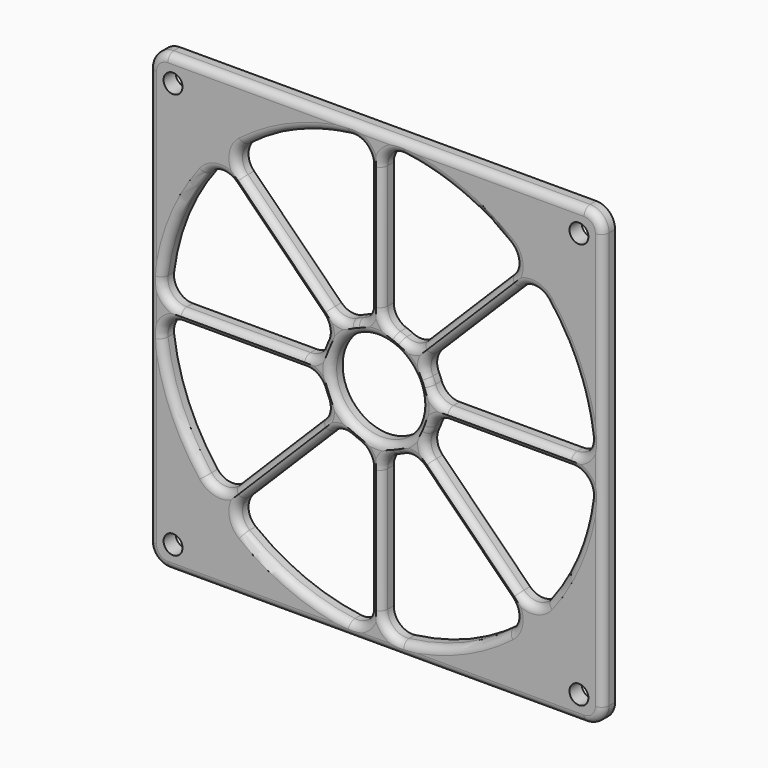
from build123d import *

# Parameters (mm, degrees)
F0_W          = 120
F0_H          = 120
F0_R          = 2.5
F0_R_2        = 12
F1_DEPTH      = 4
F2_R          = 5
F3_T1_DEPTH   = 110
F3_T3_DEPTH   = 110
F3_T5_DEPTH   = 32.6774619337
F3_T7_DEPTH   = 32.6778419819
F3_T9_DEPTH   = 32.6774619337
F3_T11_DEPTH  = 32.6774619337
F3_T13_DEPTH  = 32.6778419819
F3_T15_DEPTH  = 32.6778702464
F3_T17_DEPTH  = 32.677327087
F3_T19_DEPTH  = 32.677327087
F3_T21_DEPTH  = 32.6778419819
F3_T23_DEPTH  = 32.677327087
F3_T25_DEPTH  = 32.6778702464
F3_T27_DEPTH  = 32.677327087
F3_T29_DEPTH  = 32.6778419819
F3_T31_DEPTH  = 32.6778419819
F3_T33_DEPTH  = 32.677327087
F3_T38_ANGLE  = 30.6390253207
F3_T40_ANGLE  = 30.6387768547
F3_T42_ANGLE  = 30.6388811119
F3_T44_ANGLE  = 30.6390253207
F3_T46_ANGLE  = 30.6392737867
F3_T48_ANGLE  = 30.6386326459
F3_T50_ANGLE  = 30.6426556046
F3_T52_ANGLE  = 30.6407162297
F3_T54_ANGLE  = 90
F3_T56_ANGLE  = 90
F3_T58_ANGLE  = 90
F3_T60_ANGLE  = 90
F3_T62_ANGLE  = 97.1806115726
F3_T64_ANGLE  = 97.1786721977
F3_T66_ANGLE  = 71.0401082822
F3_T68_ANGLE  = 7.0749266488
F3_T70_ANGLE  = 71.0348183666
F3_T72_ANGLE  = 97.1786721977
F3_T74_ANGLE  = 97.1786721977
F3_T76_ANGLE  = 71.0401082822
F3_T78_ANGLE  = 7.0802165644
F3_T80_ANGLE  = 71.0401082822
F3_T82_ANGLE  = 97.1807557815
F3_T84_ANGLE  = 97.1806115726
F3_T86_ANGLE  = 71.0348183666
F3_T88_ANGLE  = 7.0692433778
F3_T90_ANGLE  = 71.0344250112
F3_T92_ANGLE  = 97.1779839331
F3_T94_ANGLE  = 97.1779839331
F3_T96_ANGLE  = 71.0419855849
F3_T98_ANGLE  = 7.0792128227
F3_T100_ANGLE = 71.0419855849
F3_T102_ANGLE = 97.1779839331
F3_T104_ANGLE = 97.1806115726
F3_T106_ANGLE = 71.0348183666
F3_T108_ANGLE = 7.074424778
F3_T110_ANGLE = 71.0419855849
F3_T112_ANGLE = 97.1779839331
F3_T114_ANGLE = 97.1807557815
F3_T116_ANGLE = 71.0344250112
F3_T118_ANGLE = 7.0740314225
F3_T120_ANGLE = 71.0419855849
F3_T122_ANGLE = 97.1806115726
F3_T124_ANGLE = 97.1806115726
F3_T126_ANGLE = 71.0348183666
F3_T128_ANGLE = 7.0696367332
F3_T130_ANGLE = 71.0348183666
F3_T132_ANGLE = 97.1779839331
F3_T134_ANGLE = 97.1806115726
F3_T136_ANGLE = 71.0348183666
F3_T138_ANGLE = 7.074424778
F3_T140_ANGLE = 71.0419855849


# Not quite as in the source:
# - a fillet or chamfer that OpenCascade refuses, or shapes differently, is made with other operations: its cross-section is extruded or revolved along the edge and cut away or added


with BuildPart() as f1:
    # F0 (on Front) → F1 (new body)
    with BuildSketch(Plane.XZ):
        Rectangle(F0_W, F0_H)
        with Locations((-53.6360389693, -53.6360389693)):
            Circle(F0_R, mode=Mode.SUBTRACT)
        with Locations((53.6360389693, -53.6360389693)):
            Circle(F0_R, mode=Mode.SUBTRACT)
        with Locations((-53.6360389693, 53.6360389693)):
            Circle(F0_R, mode=Mode.SUBTRACT)
        with BuildLine():
            ThreePointArc((56.9802597397, 1.5), (56.9950647213, 0.7500649435), (57, 0))
            ThreePointArc((57, 0), (56.9950655759, -0.75), (56.9802631579, -1.4998701467))
            ThreePointArc((56.9802631579, -1.4998701467), (52.6611333531, -21.8129556448), (41.3516988244, -39.2305621211))
            ThreePointArc((41.3516988244, -39.2305621211), (40.3050865276, -40.3050865276), (39.2305621211, -41.3516988244))
            ThreePointArc((39.2305621211, -41.3516988244), (21.8129556448, -52.6611333531), (1.4998701467, -56.9802631579))
            ThreePointArc((1.4998701467, -56.9802631579), (0.75, -56.9950655759), (0, -57))
            ThreePointArc((0, -57), (-0.75, -56.9950655759), (-1.4998701467, -56.9802631579))
            ThreePointArc((-1.4998701467, -56.9802631579), (-21.813762616, -52.6607990875), (-39.231829441, -41.3504964748))
            ThreePointArc((-39.231829441, -41.3504964748), (-40.3050865276, -40.3050865276), (-41.3504964748, -39.231829441))
            ThreePointArc((-41.3504964748, -39.231829441), (-52.6611333531, -21.8129556448), (-56.9803090988, -1.4981238267))
            ThreePointArc((-56.9803090988, -1.4981238267), (-56.9950770621, -0.7491266134), (-57, 0))
            ThreePointArc((-57, 0), (-56.9950647213, 0.7500649435), (-56.9802597397, 1.5))
            ThreePointArc((-56.9802597397, 1.5), (-52.6611084982, 21.81301565), (-41.3516988244, 39.2305621211))
            ThreePointArc((-41.3516988244, 39.2305621211), (-40.3050865276, 40.3050865276), (-39.2305621211, 41.3516988244))
            ThreePointArc((-39.2305621211, 41.3516988244), (-21.8129556448, 52.6611333531), (-1.4998701467, 56.9802631579))
            ThreePointArc((-1.4998701467, 56.9802631579), (-0.75, 56.9950655759), (0, 57))
            ThreePointArc((0, 57), (0.75, 56.9950655759), (1.4998701467, 56.9802631579))
            ThreePointArc((1.4998701467, 56.9802631579), (21.8129556448, 52.6611333531), (39.2305621211, 41.3516988244))
            ThreePointArc((39.2305621211, 41.3516988244), (40.3050865276, 40.3050865276), (41.3516988244, 39.2305621211))
            ThreePointArc((41.3516988244, 39.2305621211), (52.6611084982, 21.81301565), (56.9802597397, 1.5))
        make_face(mode=Mode.SUBTRACT)
        with Locations((53.6360389693, 53.6360389693)):
            Circle(F0_R, mode=Mode.SUBTRACT)
        with BuildLine():
            Line((-9.4942351923, 11.6129022261), (-39.2305621211, 41.3516988244))
            ThreePointArc((-39.2305621211, 41.3516988244), (-40.3050865276, 40.3050865276), (-41.3516988244, 39.2305621211))
            Line((-41.3516988244, 39.2305621211), (-11.6140130391, 9.4928763358))
            ThreePointArc((-11.6140130391, 9.4928763358), (-10.6072222233, 10.605981176), (-9.4942351923, 11.6129022261))
        make_face()
        with BuildLine():
            Line((11.6129022261, 9.4942351923), (41.3516988244, 39.2305621211))
            ThreePointArc((41.3516988244, 39.2305621211), (40.3050865276, 40.3050865276), (39.2305621211, 41.3516988244))
            Line((39.2305621211, 41.3516988244), (9.4928763358, 11.6140130391))
            ThreePointArc((9.4928763358, 11.6140130391), (10.605981176, 10.6072222233), (11.6129022261, 9.4942351923))
        make_face()
        with BuildLine():
            Line((0, 15), (0, 57))
            ThreePointArc((0, 57), (-0.75, 56.9950655759), (-1.4998701467, 56.9802631579))
            Line((-1.4998701467, 56.9802631579), (-1.4981238267, 14.925))
            ThreePointArc((-1.4981238267, 14.925), (-0.75, 14.9812382666), (0, 15))
        make_face()
        with BuildLine():
            Line((1.4981238267, 14.925), (1.4998701467, 56.9802631579))
            ThreePointArc((1.4998701467, 56.9802631579), (0.75, 56.9950655759), (0, 57))
            Line((0, 57), (0, 15))
            ThreePointArc((0, 15), (0.75, 14.9812382666), (1.4981238267, 14.925))
        make_face()
        with BuildLine():
            ThreePointArc((14.9248246068, -1.4998701467), (14.9811943633, -0.750876454), (15, 0))
            ThreePointArc((15, 0), (14.9811910967, 0.7509416259), (14.9248115566, 1.5))
            ThreePointArc((14.9248115566, 1.5), (13.8578321638, 5.7411225139), (11.6129022261, 9.4942351923))
            ThreePointArc((11.6129022261, 9.4942351923), (10.605981176, 10.6072222233), (9.4928763358, 11.6140130391))
            ThreePointArc((9.4928763358, 11.6140130391), (5.7394407225, 13.8585287889), (1.4981238267, 14.925))
            ThreePointArc((1.4981238267, 14.925), (0.75, 14.9812382666), (0, 15))
            ThreePointArc((0, 15), (-0.75, 14.9812382666), (-1.4981238267, 14.925))
            ThreePointArc((-1.4981238267, 14.925), (-5.7402514855, 13.8581929877), (-9.4942351923, 11.6129022261))
            ThreePointArc((-9.4942351923, 11.6129022261), (-10.6072222233, 10.605981176), (-11.6140130391, 9.4928763358))
            ThreePointArc((-11.6140130391, 9.4928763358), (-13.858168016, 5.740311772), (-14.9248115566, 1.5))
            ThreePointArc((-14.9248115566, 1.5), (-14.9811910967, 0.7509416259), (-15, 0))
            ThreePointArc((-15, 0), (-14.9812382666, -0.75), (-14.925, -1.4981238267))
            ThreePointArc((-14.925, -1.4981238267), (-13.8581929877, -5.7402514855), (-11.6129022261, -9.4942351923))
            ThreePointArc((-11.6129022261, -9.4942351923), (-10.6066017178, -10.6066017178), (-9.4942351923, -11.6129022261))
            ThreePointArc((-9.4942351923, -11.6129022261), (-5.7410622288, -13.857857139), (-1.4998701467, -14.9248246068))
            ThreePointArc((-1.4998701467, -14.9248246068), (-0.750876454, -14.9811943633), (0, -15))
            ThreePointArc((0, -15), (0.750876454, -14.9811943633), (1.4998701467, -14.9248246068))
            ThreePointArc((1.4998701467, -14.9248246068), (5.7410622288, -13.857857139), (9.4942351923, -11.6129022261))
            ThreePointArc((9.4942351923, -11.6129022261), (10.6072222233, -10.605981176), (11.6140130391, -9.4928763358))
            ThreePointArc((11.6140130391, -9.4928763358), (13.8581929877, -5.7402514855), (14.9248246068, -1.4998701467))
        make_face()
        Circle(F0_R_2, mode=Mode.SUBTRACT)
        with BuildLine():
            Line((15, 0), (57, 0))
            ThreePointArc((57, 0), (56.9950647213, 0.7500649435), (56.9802597397, 1.5))
            Line((56.9802597397, 1.5), (14.9248115566, 1.5))
            ThreePointArc((14.9248115566, 1.5), (14.9811910967, 0.7509416259), (15, 0))
        make_face()
        with BuildLine():
            ThreePointArc((56.9802631579, -1.4998701467), (56.9950655759, -0.75), (57, 0))
            Line((57, 0), (15, 0))
            ThreePointArc((15, 0), (14.9811943633, -0.750876454), (14.9248246068, -1.4998701467))
            Line((14.9248246068, -1.4998701467), (56.9802631579, -1.4998701467))
        make_face()
        with BuildLine():
            ThreePointArc((39.2305621211, -41.3516988244), (40.3050865276, -40.3050865276), (41.3516988244, -39.2305621211))
            Line((41.3516988244, -39.2305621211), (11.6140130391, -9.4928763358))
            ThreePointArc((11.6140130391, -9.4928763358), (10.6072222233, -10.605981176), (9.4942351923, -11.6129022261))
            Line((9.4942351923, -11.6129022261), (39.2305621211, -41.3516988244))
        make_face()
        with BuildLine():
            ThreePointArc((0, -57), (0.75, -56.9950655759), (1.4998701467, -56.9802631579))
            Line((1.4998701467, -56.9802631579), (1.4998701467, -14.9248246068))
            ThreePointArc((1.4998701467, -14.9248246068), (0.750876454, -14.9811943633), (0, -15))
            Line((0, -15), (0, -57))
        make_face()
        with BuildLine():
            ThreePointArc((-1.4998701467, -56.9802631579), (-0.75, -56.9950655759), (0, -57))
            Line((0, -57), (0, -15))
            ThreePointArc((0, -15), (-0.750876454, -14.9811943633), (-1.4998701467, -14.9248246068))
            Line((-1.4998701467, -14.9248246068), (-1.4998701467, -56.9802631579))
        make_face()
        with BuildLine():
            ThreePointArc((-41.3504964748, -39.231829441), (-40.3050865276, -40.3050865276), (-39.231829441, -41.3504964748))
            Line((-39.231829441, -41.3504964748), (-9.4942351923, -11.6129022261))
            ThreePointArc((-9.4942351923, -11.6129022261), (-10.6066017178, -10.6066017178), (-11.6129022261, -9.4942351923))
            Line((-11.6129022261, -9.4942351923), (-41.3504964748, -39.231829441))
        make_face()
        with BuildLine():
            ThreePointArc((-57, 0), (-56.9950770621, -0.7491266134), (-56.9803090988, -1.4981238267))
            Line((-56.9803090988, -1.4981238267), (-14.925, -1.4981238267))
            ThreePointArc((-14.925, -1.4981238267), (-14.9812382666, -0.75), (-15, 0))
            Line((-15, 0), (-57, 0))
        make_face()
        with BuildLine():
            Line((-14.9248115566, 1.5), (-56.9802597397, 1.5))
            ThreePointArc((-56.9802597397, 1.5), (-56.9950647213, 0.7500649435), (-57, 0))
            Line((-57, 0), (-15, 0))
            ThreePointArc((-15, 0), (-14.9811910967, 0.7509416259), (-14.9248115566, 1.5))
        make_face()
    extrude(amount=F1_DEPTH)

    # F2
    f2_edges = [f1.edges().sort_by_distance(p)[0] for p in [
        (-60, -2, 60),
        (60, -2, 60),
        (60, -2, -60),
        (-60, -2, -60),
        (-14.924812, -2, 1.5),
        (-11.614013, -2, 9.492876),
        (-9.494235, -2, 11.612902),
        (-1.498124, -2, 14.925),
        (-39.230562, -2, 41.351699),
        (-41.351699, -2, 39.230562),
        (-56.98026, -2, 1.5),
        (-56.980309, -2, -1.498124),
        (-41.350496, -2, -39.231829),
        (-14.925, -2, -1.498124),
        (-11.612902, -2, -9.494235),
        (-9.494235, -2, -11.612902),
        (-39.231829, -2, -41.350496),
        (-1.49987, -2, -56.980263),
        (-1.49987, -2, -14.924825),
        (1.49987, -2, -14.924825),
        (1.49987, -2, -56.980263),
        (39.230562, -2, -41.351699),
        (9.494235, -2, -11.612902),
        (11.614013, -2, -9.492876),
        (41.351699, -2, -39.230562),
        (56.980263, -2, -1.49987),
        (14.924825, -2, -1.49987),
        (14.924812, -2, 1.5),
        (56.98026, -2, 1.5),
        (41.351699, -2, 39.230562),
        (11.612902, -2, 9.494235),
        (9.492876, -2, 11.614013),
        (1.498124, -2, 14.925),
        (39.230562, -2, 41.351699),
        (1.49987, -2, 56.980263),
        (-1.49987, -2, 56.980263),
    ]]
    fillet(f2_edges, radius=F2_R)

    # F3: fillet of radius 2 on 10 edges, made by hand

    # F3_s2 → F3_t1 (cut)
    with BuildSketch(Plane.YZ.offset(-55)):
        with BuildLine():
            ThreePointArc((-2, 60), (-3.4142135624, 59.4142135624), (-4, 58))
            Line((-4, 58), (-4.04, 58))
            Line((-4.04, 58), (-4.04, 60.04))
            Line((-4.04, 60.04), (-2, 60.04))
            Line((-2, 60.04), (-2, 60))
        make_face()
        with BuildLine():
            ThreePointArc((-4, -58), (-3.4142135624, -59.4142135624), (-2, -60))
            Line((-2, -60), (-2, -60.04))
            Line((-2, -60.04), (-4.04, -60.04))
            Line((-4.04, -60.04), (-4.04, -58))
            Line((-4.04, -58), (-4, -58))
        make_face()
    extrude(amount=F3_T1_DEPTH, mode=Mode.SUBTRACT)

    # F3_s4 → F3_t3 (cut)
    with BuildSketch(Plane.XY.offset(-55)):
        with BuildLine():
            ThreePointArc((-58, -4), (-59.4142135624, -3.4142135624), (-60, -2))
            Line((-60, -2), (-60.04, -2))
            Line((-60.04, -2), (-60.04, -4.04))
            Line((-60.04, -4.04), (-58, -4.04))
            Line((-58, -4.04), (-58, -4))
        make_face()
        with BuildLine():
            ThreePointArc((58, -4), (59.4142135624, -3.4142135624), (60, -2))
            Line((60, -2), (60.04, -2))
            Line((60.04, -2), (60.04, -4.04))
            Line((60.04, -4.04), (58, -4.04))
            Line((58, -4.04), (58, -4))
        make_face()
    extrude(amount=F3_T3_DEPTH, mode=Mode.SUBTRACT)

    # F3_s6 → F3_t5 (cut)
    with BuildSketch(Plane(origin=(-36.4813266393, 0, -36.4813266393), x_dir=(0, 1, 0), z_dir=(0.7071067812, 0, 0.7071067812))):
        with BuildLine():
            ThreePointArc((-4, 0.5018761733), (-3.4142135624, -0.912337389), (-2, -1.4981238267))
            Line((-2, -1.4981238267), (-2, -1.5381238267))
            Line((-2, -1.5381238267), (-4.04, -1.5381238267))
            Line((-4.04, -1.5381238267), (-4.04, 0.5018761733))
            Line((-4.04, 0.5018761733), (-4, 0.5018761733))
        make_face()
    extrude(amount=F3_T5_DEPTH, mode=Mode.SUBTRACT)

    # F3_s8 → F3_t7 (cut)
    with BuildSketch(Plane.XY.offset(-51.5921669256)):
        with BuildLine():
            ThreePointArc((0.5001298533, -4), (-0.9140837091, -3.4142135624), (-1.4998701467, -2))
            Line((-1.4998701467, -2), (-1.5398701467, -2))
            Line((-1.5398701467, -2), (-1.5398701467, -4.04))
            Line((-1.5398701467, -4.04), (0.5001298533, -4.04))
            Line((0.5001298533, -4.04), (0.5001298533, -4))
        make_face()
        with BuildLine():
            ThreePointArc((-0.5001298533, -4), (0.9140837091, -3.4142135624), (1.4998701467, -2))
            Line((1.4998701467, -2), (1.5398701467, -2))
            Line((1.5398701467, -2), (1.5398701467, -4.04))
            Line((1.5398701467, -4.04), (-0.5001298533, -4.04))
            Line((-0.5001298533, -4.04), (-0.5001298533, -4))
        make_face()
    extrude(amount=F3_T7_DEPTH, mode=Mode.SUBTRACT)

    # F3_s10 → F3_t9 (cut)
    with BuildSketch(Plane.YZ.offset(-51.5923869067)):
        with BuildLine():
            ThreePointArc((-4, 0.5018761733), (-3.4142135624, -0.912337389), (-2, -1.4981238267))
            Line((-2, -1.4981238267), (-2, -1.5381238267))
            Line((-2, -1.5381238267), (-4.04, -1.5381238267))
            Line((-4.04, -1.5381238267), (-4.04, 0.5018761733))
            Line((-4.04, 0.5018761733), (-4, 0.5018761733))
        make_face()
    extrude(amount=F3_T9_DEPTH, mode=Mode.SUBTRACT)

    # F3_s12 → F3_t11 (cut)
    with BuildSketch(Plane(origin=(-13.374871714, 0, -13.374871714), x_dir=(0, 1, 0), z_dir=(-0.7071067812, 0, -0.7071067812))):
        with BuildLine():
            ThreePointArc((-4, 0.5018761733), (-3.4142135624, -0.912337389), (-2, -1.4981238267))
            Line((-2, -1.4981238267), (-2, -1.5381238267))
            Line((-2, -1.5381238267), (-4.04, -1.5381238267))
            Line((-4.04, -1.5381238267), (-4.04, 0.5018761733))
            Line((-4.04, 0.5018761733), (-4, 0.5018761733))
        make_face()
    extrude(amount=F3_T11_DEPTH, mode=Mode.SUBTRACT)

    # F3_s14 → F3_t13 (cut)
    with BuildSketch(Plane(origin=(-36.4811710892, 0, 36.4811710892), x_dir=(0, 1, 0), z_dir=(0.7071067812, 0, -0.7071067812))):
        with BuildLine():
            ThreePointArc((-4, 0.5001298533), (-3.4142135624, -0.9140837091), (-2, -1.4998701467))
            Line((-2, -1.4998701467), (-2, -1.5398701467))
            Line((-2, -1.5398701467), (-4.04, -1.5398701467))
            Line((-4.04, -1.5398701467), (-4.04, 0.5001298533))
            Line((-4.04, 0.5001298533), (-4, 0.5001298533))
        make_face()
    extrude(amount=F3_T13_DEPTH, mode=Mode.SUBTRACT)

    # F3_s16 → F3_t15 (cut)
    with BuildSketch(Plane.YZ.offset(-51.5921505658)):
        with BuildLine():
            ThreePointArc((-4, -0.5), (-3.4142135624, 0.9142135624), (-2, 1.5))
            Line((-2, 1.5), (-2, 1.54))
            Line((-2, 1.54), (-4.04, 1.54))
            Line((-4.04, 1.54), (-4.04, -0.5))
            Line((-4.04, -0.5), (-4, -0.5))
        make_face()
    extrude(amount=F3_T15_DEPTH, mode=Mode.SUBTRACT)

    # F3_s18 → F3_t17 (cut)
    with BuildSketch(Plane(origin=(-0.0021423468, 0, 51.5924649171), x_dir=(0, 1, 0), z_dir=(4.15244e-05, 0, -0.9999999991))):
        with BuildLine():
            ThreePointArc((-4, 0.5024959265), (-3.4142135624, -0.9117176359), (-2, -1.4975040735))
            Line((-2, -1.4975040735), (-2, -1.5375040735))
            Line((-2, -1.5375040735), (-4.04, -1.5375040735))
            Line((-4.04, -1.5375040735), (-4.04, 0.5024959265))
            Line((-4.04, 0.5024959265), (-4, 0.5024959265))
        make_face()
    extrude(amount=F3_T17_DEPTH, mode=Mode.SUBTRACT)

    # F3_s20 → F3_t19 (cut)
    with BuildSketch(Plane(origin=(-13.3744668567, 0, 13.3755776366), x_dir=(0, 1, 0), z_dir=(-0.7070774184, 0, 0.7071361428))):
        with BuildLine():
            ThreePointArc((-4, 0.5024959265), (-3.4142135624, -0.9117176359), (-2, -1.4975040735))
            Line((-2, -1.4975040735), (-2, -1.5375040735))
            Line((-2, -1.5375040735), (-4.04, -1.5375040735))
            Line((-4.04, -1.5375040735), (-4.04, 0.5024959265))
            Line((-4.04, 0.5024959265), (-4, 0.5024959265))
        make_face()
    extrude(amount=F3_T19_DEPTH, mode=Mode.SUBTRACT)

    # F3_s22 → F3_t21 (cut)
    with BuildSketch(Plane(origin=(36.4811710892, 0, 36.4811710892), x_dir=(0, 1, 0), z_dir=(-0.7071067812, 0, -0.7071067812))):
        with BuildLine():
            ThreePointArc((-4, 0.5001298533), (-3.4142135624, -0.9140837091), (-2, -1.4998701467))
            Line((-2, -1.4998701467), (-2, -1.5398701467))
            Line((-2, -1.5398701467), (-4.04, -1.5398701467))
            Line((-4.04, -1.5398701467), (-4.04, 0.5001298533))
            Line((-4.04, 0.5001298533), (-4, 0.5001298533))
        make_face()
    extrude(amount=F3_T21_DEPTH, mode=Mode.SUBTRACT)

    # F3_s24 → F3_t23 (cut)
    with BuildSketch(Plane(origin=(0.00078544, 0, 18.9151378583), x_dir=(0, 1, 0), z_dir=(4.15244e-05, 0, 0.9999999991))):
        with BuildLine():
            ThreePointArc((-4, 0.5024959265), (-3.4142135624, -0.9117176359), (-2, -1.4975040735))
            Line((-2, -1.4975040735), (-2, -1.5375040735))
            Line((-2, -1.5375040735), (-4.04, -1.5375040735))
            Line((-4.04, -1.5375040735), (-4.04, 0.5024959265))
            Line((-4.04, 0.5024959265), (-4, 0.5024959265))
        make_face()
    extrude(amount=F3_T23_DEPTH, mode=Mode.SUBTRACT)

    # F3_s26 → F3_t25 (cut)
    with BuildSketch(Plane.YZ.offset(18.9142803194)):
        with BuildLine():
            ThreePointArc((-4, -0.5), (-3.4142135624, 0.9142135624), (-2, 1.5))
            Line((-2, 1.5), (-2, 1.54))
            Line((-2, 1.54), (-4.04, 1.54))
            Line((-4.04, 1.54), (-4.04, -0.5))
            Line((-4.04, -0.5), (-4, -0.5))
        make_face()
    extrude(amount=F3_T25_DEPTH, mode=Mode.SUBTRACT)

    # F3_s28 → F3_t27 (cut)
    with BuildSketch(Plane(origin=(13.3755776366, 0, 13.3744668567), x_dir=(0, 1, 0), z_dir=(0.7071361428, 0, 0.7070774184))):
        with BuildLine():
            ThreePointArc((-4, 0.5024959265), (-3.4142135624, -0.9117176359), (-2, -1.4975040735))
            Line((-2, -1.4975040735), (-2, -1.5375040735))
            Line((-2, -1.5375040735), (-4.04, -1.5375040735))
            Line((-4.04, -1.5375040735), (-4.04, 0.5024959265))
            Line((-4.04, 0.5024959265), (-4, 0.5024959265))
        make_face()
    extrude(amount=F3_T27_DEPTH, mode=Mode.SUBTRACT)

    # F3_s30 → F3_t29 (cut)
    with BuildSketch(Plane(origin=(36.4811710892, 0, -36.4811710892), x_dir=(0, 1, 0), z_dir=(-0.7071067812, 0, 0.7071067812))):
        with BuildLine():
            ThreePointArc((-4, 0.5001298533), (-3.4142135624, -0.9140837091), (-2, -1.4998701467))
            Line((-2, -1.4998701467), (-2, -1.5398701467))
            Line((-2, -1.5398701467), (-4.04, -1.5398701467))
            Line((-4.04, -1.5398701467), (-4.04, 0.5001298533))
            Line((-4.04, 0.5001298533), (-4, 0.5001298533))
        make_face()
    extrude(amount=F3_T29_DEPTH, mode=Mode.SUBTRACT)

    # F3_s32 → F3_t31 (cut)
    with BuildSketch(Plane.YZ.offset(18.9143249437)):
        with BuildLine():
            ThreePointArc((-4, 0.5001298533), (-3.4142135624, -0.9140837091), (-2, -1.4998701467))
            Line((-2, -1.4998701467), (-2, -1.5398701467))
            Line((-2, -1.5398701467), (-4.04, -1.5398701467))
            Line((-4.04, -1.5398701467), (-4.04, 0.5001298533))
            Line((-4.04, 0.5001298533), (-4, 0.5001298533))
        make_face()
    extrude(amount=F3_T31_DEPTH, mode=Mode.SUBTRACT)

    # F3_s34 → F3_t33 (cut)
    with BuildSketch(Plane(origin=(13.3744668567, 0, -13.3755776366), x_dir=(0, 1, 0), z_dir=(0.7070774184, 0, -0.7071361428))):
        with BuildLine():
            ThreePointArc((-4, 0.5024959265), (-3.4142135624, -0.9117176359), (-2, -1.4975040735))
            Line((-2, -1.4975040735), (-2, -1.5375040735))
            Line((-2, -1.5375040735), (-4.04, -1.5375040735))
            Line((-4.04, -1.5375040735), (-4.04, 0.5024959265))
            Line((-4.04, 0.5024959265), (-4, 0.5024959265))
        make_face()
    extrude(amount=F3_T33_DEPTH, mode=Mode.SUBTRACT)

    # F3_s35 → F3_t36 (revolve, cut)
    with BuildSketch(Plane.XY):
        with BuildLine():
            ThreePointArc((14, -4), (12.5857864376, -3.4142135624), (12, -2))
            Line((12, -2), (11.96, -2))
            Line((11.96, -2), (11.96, -4.04))
            Line((11.96, -4.04), (14, -4.04))
            Line((14, -4.04), (14, -4))
        make_face()
    revolve(axis=Axis((0, -4, 0), (0, -1, 0)), mode=Mode.SUBTRACT)

    # F3_s37 → F3_t38 (revolve, cut)
    with BuildSketch(Plane(origin=(0, 0, 0), x_dir=(0, 1, 0), z_dir=(0.7899449053, 0, 0.6131778262))):
        with BuildLine():
            ThreePointArc((-4, -59), (-3.4142135624, -57.5857864376), (-2, -57))
            Line((-2, -57), (-2, -56.96))
            Line((-2, -56.96), (-4.04, -56.96))
            Line((-4.04, -56.96), (-4.04, -59))
            Line((-4.04, -59), (-4, -59))
        make_face()
    revolve(axis=Axis((0, -4, 0), (0, 1, 0)), revolution_arc=F3_T38_ANGLE, mode=Mode.SUBTRACT)

    # F3_s39 → F3_t40 (revolve, cut)
    with BuildSketch(Plane(origin=(0, 0, 0), x_dir=(0, 1, 0), z_dir=(0.1249975028, 0, 0.9921570563))):
        with BuildLine():
            ThreePointArc((-4, -59), (-3.4142135624, -57.5857864376), (-2, -57))
            Line((-2, -57), (-2, -56.96))
            Line((-2, -56.96), (-4.04, -56.96))
            Line((-4.04, -56.96), (-4.04, -59))
            Line((-4.04, -59), (-4, -59))
        make_face()
    revolve(axis=Axis((0, -4, 0), (0, 1, 0)), revolution_arc=F3_T40_ANGLE, mode=Mode.SUBTRACT)

    # F3_s41 → F3_t42 (revolve, cut)
    with BuildSketch(Plane(origin=(0, 0, 0), x_dir=(0, 1, 0), z_dir=(-0.6131778262, 0, 0.7899449053))):
        with BuildLine():
            ThreePointArc((-4, -59), (-3.4142135624, -57.5857864376), (-2, -57))
            Line((-2, -57), (-2, -56.96))
            Line((-2, -56.96), (-4.04, -56.96))
            Line((-4.04, -56.96), (-4.04, -59))
            Line((-4.04, -59), (-4, -59))
        make_face()
    revolve(axis=Axis((0, -4, 0), (0, 1, 0)), revolution_arc=F3_T42_ANGLE, mode=Mode.SUBTRACT)

    # F3_s43 → F3_t44 (revolve, cut)
    with BuildSketch(Plane(origin=(0, 0, 0), x_dir=(0, 1, 0), z_dir=(-0.9921575983, 0, 0.1249932003))):
        with BuildLine():
            ThreePointArc((-4, -59), (-3.4142135624, -57.5857864376), (-2, -57))
            Line((-2, -57), (-2, -56.96))
            Line((-2, -56.96), (-4.04, -56.96))
            Line((-4.04, -56.96), (-4.04, -59))
            Line((-4.04, -59), (-4, -59))
        make_face()
    revolve(axis=Axis((0, -4, 0), (0, 1, 0)), revolution_arc=F3_T44_ANGLE, mode=Mode.SUBTRACT)

    # F3_s45 → F3_t46 (revolve, cut)
    with BuildSketch(Plane(origin=(0, 0, 0), x_dir=(0, 1, 0), z_dir=(-0.7899449053, 0, -0.6131778262))):
        with BuildLine():
            ThreePointArc((-4, -59), (-3.4142135624, -57.5857864376), (-2, -57))
            Line((-2, -57), (-2, -56.96))
            Line((-2, -56.96), (-4.04, -56.96))
            Line((-4.04, -56.96), (-4.04, -59))
            Line((-4.04, -59), (-4, -59))
        make_face()
    revolve(axis=Axis((0, -4, 0), (0, 1, 0)), revolution_arc=F3_T46_ANGLE, mode=Mode.SUBTRACT)

    # F3_s47 → F3_t48 (revolve, cut)
    with BuildSketch(Plane(origin=(0, 0, 0), x_dir=(0, 1, 0), z_dir=(-0.125, 0, -0.9921567416))):
        with BuildLine():
            ThreePointArc((-4, -59), (-3.4142135624, -57.5857864376), (-2, -57))
            Line((-2, -57), (-2, -56.96))
            Line((-2, -56.96), (-4.04, -56.96))
            Line((-4.04, -56.96), (-4.04, -59))
            Line((-4.04, -59), (-4, -59))
        make_face()
    revolve(axis=Axis((0, -4, 0), (0, 1, 0)), revolution_arc=F3_T48_ANGLE, mode=Mode.SUBTRACT)

    # F3_s49 → F3_t50 (revolve, cut)
    with BuildSketch(Plane(origin=(0, 0, 0), x_dir=(0, 1, 0), z_dir=(0.6132011388, 0, -0.7899268089))):
        with BuildLine():
            ThreePointArc((-4, -59), (-3.4142135624, -57.5857864376), (-2, -57))
            Line((-2, -57), (-2, -56.96))
            Line((-2, -56.96), (-4.04, -56.96))
            Line((-4.04, -56.96), (-4.04, -59))
            Line((-4.04, -59), (-4, -59))
        make_face()
    revolve(axis=Axis((0, -4, 0), (0, 1, 0)), revolution_arc=F3_T50_ANGLE, mode=Mode.SUBTRACT)

    # F3_s51 → F3_t52 (revolve, cut)
    with BuildSketch(Plane(origin=(0, 0, 0), x_dir=(0, 1, 0), z_dir=(0.9921570563, 0, -0.1249975028))):
        with BuildLine():
            ThreePointArc((-4, -59), (-3.4142135624, -57.5857864376), (-2, -57))
            Line((-2, -57), (-2, -56.96))
            Line((-2, -56.96), (-4.04, -56.96))
            Line((-4.04, -56.96), (-4.04, -59))
            Line((-4.04, -59), (-4, -59))
        make_face()
    revolve(axis=Axis((0, -4, 0), (0, 1, 0)), revolution_arc=F3_T52_ANGLE, mode=Mode.SUBTRACT)

    # F3_s53 → F3_t54 (revolve, cut)
    with BuildSketch(Plane.YZ.offset(55)):
        with BuildLine():
            ThreePointArc((-2, 60), (-3.4142135624, 59.4142135624), (-4, 58))
            Line((-4, 58), (-4.04, 58))
            Line((-4.04, 58), (-4.04, 60.04))
            Line((-4.04, 60.04), (-2, 60.04))
            Line((-2, 60.04), (-2, 60))
        make_face()
    revolve(axis=Axis((55, -4, 55), (0, 1, 0)), revolution_arc=F3_T54_ANGLE, mode=Mode.SUBTRACT)

    # F3_s55 → F3_t56 (revolve, cut)
    with BuildSketch(Plane.YZ.offset(-55)):
        with BuildLine():
            ThreePointArc((-2, 60), (-3.4142135624, 59.4142135624), (-4, 58))
            Line((-4, 58), (-4.04, 58))
            Line((-4.04, 58), (-4.04, 60.04))
            Line((-4.04, 60.04), (-2, 60.04))
            Line((-2, 60.04), (-2, 60))
        make_face()
    revolve(axis=Axis((-55, -4, 55), (0, -1, 0)), revolution_arc=F3_T56_ANGLE, mode=Mode.SUBTRACT)

    # F3_s57 → F3_t58 (revolve, cut)
    with BuildSketch(Plane.XY.offset(-55)):
        with BuildLine():
            ThreePointArc((-58, -4), (-59.4142135624, -3.4142135624), (-60, -2))
            Line((-60, -2), (-60.04, -2))
            Line((-60.04, -2), (-60.04, -4.04))
            Line((-60.04, -4.04), (-58, -4.04))
            Line((-58, -4.04), (-58, -4))
        make_face()
    revolve(axis=Axis((-55, -4, -55), (0, -1, 0)), revolution_arc=F3_T58_ANGLE, mode=Mode.SUBTRACT)

    # F3_s59 → F3_t60 (revolve, cut)
    with BuildSketch(Plane.YZ.offset(55)):
        with BuildLine():
            ThreePointArc((-4, -58), (-3.4142135624, -59.4142135624), (-2, -60))
            Line((-2, -60), (-2, -60.04))
            Line((-2, -60.04), (-4.04, -60.04))
            Line((-4.04, -60.04), (-4.04, -58))
            Line((-4.04, -58), (-4, -58))
        make_face()
    revolve(axis=Axis((55, -4, -55), (0, -1, 0)), revolution_arc=F3_T60_ANGLE, mode=Mode.SUBTRACT)

    # F3_s61 → F3_t62 (revolve, cut)
    with BuildSketch(Plane.XY.offset(-51.5921669256)):
        with BuildLine():
            ThreePointArc((0.5001298533, -4), (-0.9140837091, -3.4142135624), (-1.4998701467, -2))
            Line((-1.4998701467, -2), (-1.5398701467, -2))
            Line((-1.5398701467, -2), (-1.5398701467, -4.04))
            Line((-1.5398701467, -4.04), (0.5001298533, -4.04))
            Line((0.5001298533, -4.04), (0.5001298533, -4))
        make_face()
    revolve(axis=Axis((-6.4998701467, -4, -51.5921669256), (0, 1, 0)), revolution_arc=F3_T62_ANGLE, mode=Mode.SUBTRACT)

    # F3_s63 → F3_t64 (revolve, cut)
    with BuildSketch(Plane(origin=(0, 0, 0), x_dir=(0, 1, 0), z_dir=(0.7899268089, 0, -0.6132011388))):
        with BuildLine():
            ThreePointArc((-4, -59), (-3.4142135624, -57.5857864376), (-2, -57))
            Line((-2, -57), (-2, -56.96))
            Line((-2, -56.96), (-4.04, -56.96))
            Line((-4.04, -56.96), (-4.04, -59))
            Line((-4.04, -59), (-4, -59))
        make_face()
    revolve(axis=Axis((-31.8864592165, -4, -41.0761940622), (0, 1, 0)), revolution_arc=F3_T64_ANGLE, mode=Mode.SUBTRACT)

    # F3_s65 → F3_t66 (revolve, cut)
    with BuildSketch(Plane(origin=(0, 0, 0), x_dir=(0, 1, 0), z_dir=(0.8984869568, 0, -0.4390002146))):
        with BuildLine():
            ThreePointArc((-4, -13), (-3.4142135624, -14.4142135624), (-2, -15))
            Line((-2, -15), (-2, -15.04))
            Line((-2, -15.04), (-4.04, -15.04))
            Line((-4.04, -15.04), (-4.04, -13))
            Line((-4.04, -13), (-4, -13))
        make_face()
    revolve(axis=Axis((-8.7800042912, -4, -17.9697391368), (0, -1, 0)), revolution_arc=F3_T66_ANGLE, mode=Mode.SUBTRACT)

    # F3_s67 → F3_t68 (revolve, cut)
    with BuildSketch(Plane(origin=(0, 0, 0), x_dir=(0, 1, 0), z_dir=(-0.8984869568, 0, 0.4390002146))):
        with BuildLine():
            ThreePointArc((-4, 13), (-3.4142135624, 14.4142135624), (-2, 15))
            Line((-2, 15), (-2, 15.04))
            Line((-2, 15.04), (-4.04, 15.04))
            Line((-4.04, 15.04), (-4.04, 13))
            Line((-4.04, 13), (-4, 13))
        make_face()
    revolve(axis=Axis((0, -4, 0), (0, -1, 0)), revolution_arc=F3_T68_ANGLE, mode=Mode.SUBTRACT)

    # F3_s69 → F3_t70 (revolve, cut)
    with BuildSketch(Plane(origin=(0, 0, 0), x_dir=(0, 1, 0), z_dir=(-0.9457162472, 0, 0.3249935073))):
        with BuildLine():
            ThreePointArc((-4, 13), (-3.4142135624, 14.4142135624), (-2, 15))
            Line((-2, 15), (-2, 15.04))
            Line((-2, 15.04), (-4.04, 15.04))
            Line((-4.04, 15.04), (-4.04, 13))
            Line((-4.04, 13), (-4, 13))
        make_face()
    revolve(axis=Axis((-6.4998701467, -4, -18.9143249437), (0, 1, 0)), revolution_arc=F3_T70_ANGLE, mode=Mode.SUBTRACT)

    # F3_s71 → F3_t72 (revolve, cut)
    with BuildSketch(Plane(origin=(-36.4813266393, 0, -36.4813266393), x_dir=(0, 1, 0), z_dir=(0.7071067812, 0, 0.7071067812))):
        with BuildLine():
            ThreePointArc((-4, -0.5018761733), (-3.4142135624, 0.912337389), (-2, 1.4981238267))
            Line((-2, 1.4981238267), (-2, 1.5381238267))
            Line((-2, 1.5381238267), (-4.04, 1.5381238267))
            Line((-4.04, 1.5381238267), (-4.04, -0.5018761733))
            Line((-4.04, -0.5018761733), (-4, -0.5018761733))
        make_face()
    revolve(axis=Axis((-41.0761940622, -4, -31.8864592165), (0, 1, 0)), revolution_arc=F3_T72_ANGLE, mode=Mode.SUBTRACT)

    # F3_s73 → F3_t74 (revolve, cut)
    with BuildSketch(Plane(origin=(0, 0, 0), x_dir=(0, 1, 0), z_dir=(0.1249639197, 0, -0.9921612867))):
        with BuildLine():
            ThreePointArc((-4, -59), (-3.4142135624, -57.5857864376), (-2, -57))
            Line((-2, -57), (-2, -56.96))
            Line((-2, -56.96), (-4.04, -56.96))
            Line((-4.04, -56.96), (-4.04, -59))
            Line((-4.04, -59), (-4, -59))
        make_face()
    revolve(axis=Axis((-51.5923869067, -4, -6.4981238267), (0, 1, 0)), revolution_arc=F3_T74_ANGLE, mode=Mode.SUBTRACT)

    # F3_s75 → F3_t76 (revolve, cut)
    with BuildSketch(Plane(origin=(0, 0, 0), x_dir=(0, 1, 0), z_dir=(0.3249061913, 0, -0.9457462486))):
        with BuildLine():
            ThreePointArc((-4, -13), (-3.4142135624, -14.4142135624), (-2, -15))
            Line((-2, -15), (-2, -15.04))
            Line((-2, -15.04), (-4.04, -15.04))
            Line((-4.04, -15.04), (-4.04, -13))
            Line((-4.04, -13), (-4, -13))
        make_face()
    revolve(axis=Axis((-18.914924973, -4, -6.4981238267), (0, -1, 0)), revolution_arc=F3_T76_ANGLE, mode=Mode.SUBTRACT)

    # F3_s77 → F3_t78 (revolve, cut)
    with BuildSketch(Plane(origin=(0, 0, 0), x_dir=(0, 1, 0), z_dir=(-0.3249061913, 0, 0.9457462486))):
        with BuildLine():
            ThreePointArc((-4, 13), (-3.4142135624, 14.4142135624), (-2, 15))
            Line((-2, 15), (-2, 15.04))
            Line((-2, 15.04), (-4.04, 15.04))
            Line((-4.04, 15.04), (-4.04, 13))
            Line((-4.04, 13), (-4, 13))
        make_face()
    revolve(axis=Axis((0, -4, 0), (0, -1, 0)), revolution_arc=F3_T78_ANGLE, mode=Mode.SUBTRACT)

    # F3_s79 → F3_t80 (revolve, cut)
    with BuildSketch(Plane(origin=(0, 0, 0), x_dir=(0, 1, 0), z_dir=(-0.4390002146, 0, 0.8984869568))):
        with BuildLine():
            ThreePointArc((-4, 13), (-3.4142135624, 14.4142135624), (-2, 15))
            Line((-2, 15), (-2, 15.04))
            Line((-2, 15.04), (-4.04, 15.04))
            Line((-4.04, 15.04), (-4.04, 13))
            Line((-4.04, 13), (-4, 13))
        make_face()
    revolve(axis=Axis((-17.9697391368, -4, -8.7800042912), (0, 1, 0)), revolution_arc=F3_T80_ANGLE, mode=Mode.SUBTRACT)

    # F3_s81 → F3_t82 (revolve, cut)
    with BuildSketch(Plane.YZ.offset(-51.5921505658)):
        with BuildLine():
            ThreePointArc((-4, -0.5), (-3.4142135624, 0.9142135624), (-2, 1.5))
            Line((-2, 1.5), (-2, 1.54))
            Line((-2, 1.54), (-4.04, 1.54))
            Line((-4.04, 1.54), (-4.04, -0.5))
            Line((-4.04, -0.5), (-4, -0.5))
        make_face()
    revolve(axis=Axis((-51.5921505658, -4, 6.5), (0, 1, 0)), revolution_arc=F3_T82_ANGLE, mode=Mode.SUBTRACT)

    # F3_s83 → F3_t84 (revolve, cut)
    with BuildSketch(Plane(origin=(-36.4811710892, 0, 36.4811710892), x_dir=(0, 1, 0), z_dir=(0.7071067812, 0, -0.7071067812))):
        with BuildLine():
            ThreePointArc((-4, 0.5001298533), (-3.4142135624, -0.9140837091), (-2, -1.4998701467))
            Line((-2, -1.4998701467), (-2, -1.5398701467))
            Line((-2, -1.5398701467), (-4.04, -1.5398701467))
            Line((-4.04, -1.5398701467), (-4.04, 0.5001298533))
            Line((-4.04, 0.5001298533), (-4, 0.5001298533))
        make_face()
    revolve(axis=Axis((-41.0772733468, -4, 31.8850688316), (0, -1, 0)), revolution_arc=F3_T84_ANGLE, mode=Mode.SUBTRACT)

    # F3_s85 → F3_t86 (revolve, cut)
    with BuildSketch(Plane(origin=(-13.3744474293, 0, 13.3744474293), x_dir=(0, 1, 0), z_dir=(-0.7071067812, 0, 0.7071067812))):
        with BuildLine():
            ThreePointArc((-4, -0.5001298533), (-3.4142135624, 0.9140837091), (-2, 1.4998701467))
            Line((-2, 1.4998701467), (-2, 1.5398701467))
            Line((-2, 1.5398701467), (-4.04, 1.5398701467))
            Line((-4.04, 1.5398701467), (-4.04, -0.5001298533))
            Line((-4.04, -0.5001298533), (-4, -0.5001298533))
        make_face()
    revolve(axis=Axis((-17.9705496868, -4, 8.7783451717), (0, 1, 0)), revolution_arc=F3_T86_ANGLE, mode=Mode.SUBTRACT)

    # F3_s87 → F3_t88 (revolve, cut)
    with BuildSketch(Plane(origin=(0, 0, 0), x_dir=(0, 1, 0), z_dir=(0.4389172586, 0, 0.8985274843))):
        with BuildLine():
            ThreePointArc((-4, 13), (-3.4142135624, 14.4142135624), (-2, 15))
            Line((-2, 15), (-2, 15.04))
            Line((-2, 15.04), (-4.04, 15.04))
            Line((-4.04, 15.04), (-4.04, 13))
            Line((-4.04, 13), (-4, 13))
        make_face()
    revolve(axis=Axis((0, -4, 0), (0, -1, 0)), revolution_arc=F3_T88_ANGLE, mode=Mode.SUBTRACT)

    # F3_s89 → F3_t90 (revolve, cut)
    with BuildSketch(Plane(origin=(0, 0, 0), x_dir=(0, 1, 0), z_dir=(0.325, 0, 0.945714016))):
        with BuildLine():
            ThreePointArc((-4, 13), (-3.4142135624, 14.4142135624), (-2, 15))
            Line((-2, 15), (-2, 15.04))
            Line((-2, 15.04), (-4.04, 15.04))
            Line((-4.04, 15.04), (-4.04, 13))
            Line((-4.04, 13), (-4, 13))
        make_face()
    revolve(axis=Axis((-18.9142803194, -4, 6.5), (0, 1, 0)), revolution_arc=F3_T90_ANGLE, mode=Mode.SUBTRACT)

    # F3_s91 → F3_t92 (revolve, cut)
    with BuildSketch(Plane(origin=(-36.4798669331, 0, 36.482896669), x_dir=(0, 1, 0), z_dir=(0.7070774184, 0, -0.7071361428))):
        with BuildLine():
            ThreePointArc((-4, -0.5024959265), (-3.4142135624, 0.9117176359), (-2, 1.4975040735))
            Line((-2, 1.4975040735), (-2, 1.5375040735))
            Line((-2, 1.5375040735), (-4.04, 1.5375040735))
            Line((-4.04, 1.5375040735), (-4.04, -0.5024959265))
            Line((-4.04, -0.5024959265), (-4, -0.5024959265))
        make_face()
    revolve(axis=Axis((-31.8852469649, -4, 41.0771350752), (0, 1, 0)), revolution_arc=F3_T92_ANGLE, mode=Mode.SUBTRACT)

    # F3_s93 → F3_t94 (revolve, cut)
    with BuildSketch(Plane(origin=(0, 0, 0), x_dir=(0, 1, 0), z_dir=(-0.9921575983, 0, -0.1249932003))):
        with BuildLine():
            ThreePointArc((-4, -59), (-3.4142135624, -57.5857864376), (-2, -57))
            Line((-2, -57), (-2, -56.96))
            Line((-2, -56.96), (-4.04, -56.96))
            Line((-4.04, -56.96), (-4.04, -59))
            Line((-4.04, -59), (-4, -59))
        make_face()
    revolve(axis=Axis((-6.4996464147, -4, 51.5921951121), (0, 1, 0)), revolution_arc=F3_T94_ANGLE, mode=Mode.SUBTRACT)

    # F3_s95 → F3_t96 (revolve, cut)
    with BuildSketch(Plane(origin=(-0.00078544, 0, 18.9151378583), x_dir=(0, 1, 0), z_dir=(-4.15244e-05, 0, 0.9999999991))):
        with BuildLine():
            ThreePointArc((-4, -0.5024959265), (-3.4142135624, 0.9117176359), (-2, 1.4975040735))
            Line((-2, 1.4975040735), (-2, 1.5375040735))
            Line((-2, 1.5375040735), (-4.04, 1.5375040735))
            Line((-4.04, 1.5375040735), (-4.04, -0.5024959265))
            Line((-4.04, -0.5024959265), (-4, -0.5024959265))
        make_face()
    revolve(axis=Axis((-6.4982895079, -4, 18.9148680532), (0, 1, 0)), revolution_arc=F3_T96_ANGLE, mode=Mode.SUBTRACT)

    # F3_s97 → F3_t98 (revolve, cut)
    with BuildSketch(Plane(origin=(0, 0, 0), x_dir=(0, 1, 0), z_dir=(0.9457434027, 0, 0.3249144754))):
        with BuildLine():
            ThreePointArc((-4, 13), (-3.4142135624, 14.4142135624), (-2, 15))
            Line((-2, 15), (-2, 15.04))
            Line((-2, 15.04), (-4.04, 15.04))
            Line((-4.04, 15.04), (-4.04, 13))
            Line((-4.04, 13), (-4, 13))
        make_face()
    revolve(axis=Axis((0, -4, 0), (0, -1, 0)), revolution_arc=F3_T98_ANGLE, mode=Mode.SUBTRACT)

    # F3_s99 → F3_t100 (revolve, cut)
    with BuildSketch(Plane(origin=(-13.3744668567, 0, 13.3755776366), x_dir=(0, 1, 0), z_dir=(-0.7070774184, 0, 0.7071361428))):
        with BuildLine():
            ThreePointArc((-4, 0.5024959265), (-3.4142135624, -0.9117176359), (-2, -1.4975040735))
            Line((-2, -1.4975040735), (-2, -1.5375040735))
            Line((-2, -1.5375040735), (-4.04, -1.5375040735))
            Line((-4.04, -1.5375040735), (-4.04, 0.5024959265))
            Line((-4.04, 0.5024959265), (-4, 0.5024959265))
        make_face()
    revolve(axis=Axis((-8.7798468886, -4, 17.9698160428), (0, -1, 0)), revolution_arc=F3_T100_ANGLE, mode=Mode.SUBTRACT)

    # F3_s101 → F3_t102 (revolve, cut)
    with BuildSketch(Plane(origin=(0.0021423468, 0, 51.5924649171), x_dir=(0, 1, 0), z_dir=(-4.15244e-05, 0, -0.9999999991))):
        with BuildLine():
            ThreePointArc((-4, -0.5024959265), (-3.4142135624, 0.9117176359), (-2, 1.4975040735))
            Line((-2, 1.4975040735), (-2, 1.5375040735))
            Line((-2, 1.5375040735), (-4.04, 1.5375040735))
            Line((-4.04, 1.5375040735), (-4.04, -0.5024959265))
            Line((-4.04, -0.5024959265), (-4, -0.5024959265))
        make_face()
    revolve(axis=Axis((6.4996464147, -4, 51.5921951121), (0, 1, 0)), revolution_arc=F3_T102_ANGLE, mode=Mode.SUBTRACT)

    # F3_s103 → F3_t104 (revolve, cut)
    with BuildSketch(Plane(origin=(0, 0, 0), x_dir=(0, 1, 0), z_dir=(-0.7899475644, 0, 0.6131744006))):
        with BuildLine():
            ThreePointArc((-4, -59), (-3.4142135624, -57.5857864376), (-2, -57))
            Line((-2, -57), (-2, -56.96))
            Line((-2, -56.96), (-4.04, -56.96))
            Line((-4.04, -56.96), (-4.04, -59))
            Line((-4.04, -59), (-4, -59))
        make_face()
    revolve(axis=Axis((31.8850688316, -4, 41.0772733468), (0, 1, 0)), revolution_arc=F3_T104_ANGLE, mode=Mode.SUBTRACT)

    # F3_s105 → F3_t106 (revolve, cut)
    with BuildSketch(Plane(origin=(13.3744474293, 0, 13.3744474293), x_dir=(0, 1, 0), z_dir=(0.7071067812, 0, 0.7071067812))):
        with BuildLine():
            ThreePointArc((-4, -0.5001298533), (-3.4142135624, 0.9140837091), (-2, 1.4998701467))
            Line((-2, 1.4998701467), (-2, 1.5398701467))
            Line((-2, 1.5398701467), (-4.04, 1.5398701467))
            Line((-4.04, 1.5398701467), (-4.04, -0.5001298533))
            Line((-4.04, -0.5001298533), (-4, -0.5001298533))
        make_face()
    revolve(axis=Axis((8.7783451717, -4, 17.9705496868), (0, 1, 0)), revolution_arc=F3_T106_ANGLE, mode=Mode.SUBTRACT)

    # F3_s107 → F3_t108 (revolve, cut)
    with BuildSketch(Plane(origin=(0, 0, 0), x_dir=(0, 1, 0), z_dir=(0.8985274843, 0, -0.4389172586))):
        with BuildLine():
            ThreePointArc((-4, 13), (-3.4142135624, 14.4142135624), (-2, 15))
            Line((-2, 15), (-2, 15.04))
            Line((-2, 15.04), (-4.04, 15.04))
            Line((-4.04, 15.04), (-4.04, 13))
            Line((-4.04, 13), (-4, 13))
        make_face()
    revolve(axis=Axis((0, -4, 0), (0, -1, 0)), revolution_arc=F3_T108_ANGLE, mode=Mode.SUBTRACT)

    # F3_s109 → F3_t110 (revolve, cut)
    with BuildSketch(Plane(origin=(0.00078544, 0, 18.9151378583), x_dir=(0, 1, 0), z_dir=(4.15244e-05, 0, 0.9999999991))):
        with BuildLine():
            ThreePointArc((-4, 0.5024959265), (-3.4142135624, -0.9117176359), (-2, -1.4975040735))
            Line((-2, -1.4975040735), (-2, -1.5375040735))
            Line((-2, -1.5375040735), (-4.04, -1.5375040735))
            Line((-4.04, -1.5375040735), (-4.04, 0.5024959265))
            Line((-4.04, 0.5024959265), (-4, 0.5024959265))
        make_face()
    revolve(axis=Axis((6.4982895079, -4, 18.9148680532), (0, -1, 0)), revolution_arc=F3_T110_ANGLE, mode=Mode.SUBTRACT)

    # F3_s111 → F3_t112 (revolve, cut)
    with BuildSketch(Plane(origin=(36.482896669, 0, 36.4798669331), x_dir=(0, 1, 0), z_dir=(-0.7071361428, 0, -0.7070774184))):
        with BuildLine():
            ThreePointArc((-4, -0.5024959265), (-3.4142135624, 0.9117176359), (-2, 1.4975040735))
            Line((-2, 1.4975040735), (-2, 1.5375040735))
            Line((-2, 1.5375040735), (-4.04, 1.5375040735))
            Line((-4.04, 1.5375040735), (-4.04, -0.5024959265))
            Line((-4.04, -0.5024959265), (-4, -0.5024959265))
        make_face()
    revolve(axis=Axis((41.0771350752, -4, 31.8852469649), (0, 1, 0)), revolution_arc=F3_T112_ANGLE, mode=Mode.SUBTRACT)

    # F3_s113 → F3_t114 (revolve, cut)
    with BuildSketch(Plane(origin=(0, 0, 0), x_dir=(0, 1, 0), z_dir=(-0.125, 0, 0.9921567416))):
        with BuildLine():
            ThreePointArc((-4, -59), (-3.4142135624, -57.5857864376), (-2, -57))
            Line((-2, -57), (-2, -56.96))
            Line((-2, -56.96), (-4.04, -56.96))
            Line((-4.04, -56.96), (-4.04, -59))
            Line((-4.04, -59), (-4, -59))
        make_face()
    revolve(axis=Axis((51.5921505658, -4, 6.5), (0, 1, 0)), revolution_arc=F3_T114_ANGLE, mode=Mode.SUBTRACT)

    # F3_s115 → F3_t116 (revolve, cut)
    with BuildSketch(Plane(origin=(0, 0, 0), x_dir=(0, 1, 0), z_dir=(-0.325, 0, 0.945714016))):
        with BuildLine():
            ThreePointArc((-4, -13), (-3.4142135624, -14.4142135624), (-2, -15))
            Line((-2, -15), (-2, -15.04))
            Line((-2, -15.04), (-4.04, -15.04))
            Line((-4.04, -15.04), (-4.04, -13))
            Line((-4.04, -13), (-4, -13))
        make_face()
    revolve(axis=Axis((18.9142803194, -4, 6.5), (0, -1, 0)), revolution_arc=F3_T116_ANGLE, mode=Mode.SUBTRACT)

    # F3_s117 → F3_t118 (revolve, cut)
    with BuildSketch(Plane(origin=(0, 0, 0), x_dir=(0, 1, 0), z_dir=(0.325, 0, -0.945714016))):
        with BuildLine():
            ThreePointArc((-4, 13), (-3.4142135624, 14.4142135624), (-2, 15))
            Line((-2, 15), (-2, 15.04))
            Line((-2, 15.04), (-4.04, 15.04))
            Line((-4.04, 15.04), (-4.04, 13))
            Line((-4.04, 13), (-4, 13))
        make_face()
    revolve(axis=Axis((0, -4, 0), (0, -1, 0)), revolution_arc=F3_T118_ANGLE, mode=Mode.SUBTRACT)

    # F3_s119 → F3_t120 (revolve, cut)
    with BuildSketch(Plane(origin=(0, 0, 0), x_dir=(0, 1, 0), z_dir=(0.4389923444, 0, -0.8984908021))):
        with BuildLine():
            ThreePointArc((-4, 13), (-3.4142135624, 14.4142135624), (-2, 15))
            Line((-2, 15), (-2, 15.04))
            Line((-2, 15.04), (-4.04, 15.04))
            Line((-4.04, 15.04), (-4.04, 13))
            Line((-4.04, 13), (-4, 13))
        make_face()
    revolve(axis=Axis((17.9698160428, -4, 8.7798468886), (0, 1, 0)), revolution_arc=F3_T120_ANGLE, mode=Mode.SUBTRACT)

    # F3_s121 → F3_t122 (revolve, cut)
    with BuildSketch(Plane.YZ.offset(51.5921669256)):
        with BuildLine():
            ThreePointArc((-4, 0.5001298533), (-3.4142135624, -0.9140837091), (-2, -1.4998701467))
            Line((-2, -1.4998701467), (-2, -1.5398701467))
            Line((-2, -1.5398701467), (-4.04, -1.5398701467))
            Line((-4.04, -1.5398701467), (-4.04, 0.5001298533))
            Line((-4.04, 0.5001298533), (-4, 0.5001298533))
        make_face()
    revolve(axis=Axis((51.5921669256, -4, -6.4998701467), (0, 1, 0)), revolution_arc=F3_T122_ANGLE, mode=Mode.SUBTRACT)

    # F3_s123 → F3_t124 (revolve, cut)
    with BuildSketch(Plane(origin=(0, 0, 0), x_dir=(0, 1, 0), z_dir=(0.6131744006, 0, 0.7899475644))):
        with BuildLine():
            ThreePointArc((-4, -59), (-3.4142135624, -57.5857864376), (-2, -57))
            Line((-2, -57), (-2, -56.96))
            Line((-2, -56.96), (-4.04, -56.96))
            Line((-4.04, -56.96), (-4.04, -59))
            Line((-4.04, -59), (-4, -59))
        make_face()
    revolve(axis=Axis((41.0772733468, -4, -31.8850688316), (0, 1, 0)), revolution_arc=F3_T124_ANGLE, mode=Mode.SUBTRACT)

    # F3_s125 → F3_t126 (revolve, cut)
    with BuildSketch(Plane(origin=(0, 0, 0), x_dir=(0, 1, 0), z_dir=(0.4389172586, 0, 0.8985274843))):
        with BuildLine():
            ThreePointArc((-4, -13), (-3.4142135624, -14.4142135624), (-2, -15))
            Line((-2, -15), (-2, -15.04))
            Line((-2, -15.04), (-4.04, -15.04))
            Line((-4.04, -15.04), (-4.04, -13))
            Line((-4.04, -13), (-4, -13))
        make_face()
    revolve(axis=Axis((17.9705496868, -4, -8.7783451717), (0, -1, 0)), revolution_arc=F3_T126_ANGLE, mode=Mode.SUBTRACT)

    # F3_s127 → F3_t128 (revolve, cut)
    with BuildSketch(Plane(origin=(0, 0, 0), x_dir=(0, 1, 0), z_dir=(-0.4389172586, 0, -0.8985274843))):
        with BuildLine():
            ThreePointArc((-4, 13), (-3.4142135624, 14.4142135624), (-2, 15))
            Line((-2, 15), (-2, 15.04))
            Line((-2, 15.04), (-4.04, 15.04))
            Line((-4.04, 15.04), (-4.04, 13))
            Line((-4.04, 13), (-4, 13))
        make_face()
    revolve(axis=Axis((0, -4, 0), (0, -1, 0)), revolution_arc=F3_T128_ANGLE, mode=Mode.SUBTRACT)

    # F3_s129 → F3_t130 (revolve, cut)
    with BuildSketch(Plane(origin=(0, 0, 0), x_dir=(0, 1, 0), z_dir=(-0.3249935073, 0, -0.9457162472))):
        with BuildLine():
            ThreePointArc((-4, 13), (-3.4142135624, 14.4142135624), (-2, 15))
            Line((-2, 15), (-2, 15.04))
            Line((-2, 15.04), (-4.04, 15.04))
            Line((-4.04, 15.04), (-4.04, 13))
            Line((-4.04, 13), (-4, 13))
        make_face()
    revolve(axis=Axis((18.9143249437, -4, -6.4998701467), (0, 1, 0)), revolution_arc=F3_T130_ANGLE, mode=Mode.SUBTRACT)

    # F3_s131 → F3_t132 (revolve, cut)
    with BuildSketch(Plane(origin=(36.4798669331, 0, -36.482896669), x_dir=(0, 1, 0), z_dir=(-0.7070774184, 0, 0.7071361428))):
        with BuildLine():
            ThreePointArc((-4, -0.5024959265), (-3.4142135624, 0.9117176359), (-2, 1.4975040735))
            Line((-2, 1.4975040735), (-2, 1.5375040735))
            Line((-2, 1.5375040735), (-4.04, 1.5375040735))
            Line((-4.04, 1.5375040735), (-4.04, -0.5024959265))
            Line((-4.04, -0.5024959265), (-4, -0.5024959265))
        make_face()
    revolve(axis=Axis((31.8852469649, -4, -41.0771350752), (0, 1, 0)), revolution_arc=F3_T132_ANGLE, mode=Mode.SUBTRACT)

    # F3_s133 → F3_t134 (revolve, cut)
    with BuildSketch(Plane(origin=(0, 0, 0), x_dir=(0, 1, 0), z_dir=(0.9921570563, 0, 0.1249975028))):
        with BuildLine():
            ThreePointArc((-4, -59), (-3.4142135624, -57.5857864376), (-2, -57))
            Line((-2, -57), (-2, -56.96))
            Line((-2, -56.96), (-4.04, -56.96))
            Line((-4.04, -56.96), (-4.04, -59))
            Line((-4.04, -59), (-4, -59))
        make_face()
    revolve(axis=Axis((6.4998701467, -4, -51.5921669256), (0, 1, 0)), revolution_arc=F3_T134_ANGLE, mode=Mode.SUBTRACT)

    # F3_s135 → F3_t136 (revolve, cut)
    with BuildSketch(Plane(origin=(0, 0, 0), x_dir=(0, 1, 0), z_dir=(0.9457162472, 0, 0.3249935073))):
        with BuildLine():
            ThreePointArc((-4, -13), (-3.4142135624, -14.4142135624), (-2, -15))
            Line((-2, -15), (-2, -15.04))
            Line((-2, -15.04), (-4.04, -15.04))
            Line((-4.04, -15.04), (-4.04, -13))
            Line((-4.04, -13), (-4, -13))
        make_face()
    revolve(axis=Axis((6.4998701467, -4, -18.9143249437), (0, -1, 0)), revolution_arc=F3_T136_ANGLE, mode=Mode.SUBTRACT)

    # F3_s137 → F3_t138 (revolve, cut)
    with BuildSketch(Plane(origin=(0, 0, 0), x_dir=(0, 1, 0), z_dir=(-0.9457162472, 0, -0.3249935073))):
        with BuildLine():
            ThreePointArc((-4, 13), (-3.4142135624, 14.4142135624), (-2, 15))
            Line((-2, 15), (-2, 15.04))
            Line((-2, 15.04), (-4.04, 15.04))
            Line((-4.04, 15.04), (-4.04, 13))
            Line((-4.04, 13), (-4, 13))
        make_face()
    revolve(axis=Axis((0, -4, 0), (0, -1, 0)), revolution_arc=F3_T138_ANGLE, mode=Mode.SUBTRACT)

    # F3_s139 → F3_t140 (revolve, cut)
    with BuildSketch(Plane(origin=(0, 0, 0), x_dir=(0, 1, 0), z_dir=(-0.8984908021, 0, -0.4389923444))):
        with BuildLine():
            ThreePointArc((-4, 13), (-3.4142135624, 14.4142135624), (-2, 15))
            Line((-2, 15), (-2, 15.04))
            Line((-2, 15.04), (-4.04, 15.04))
            Line((-4.04, 15.04), (-4.04, 13))
            Line((-4.04, 13), (-4, 13))
        make_face()
    revolve(axis=Axis((8.7798468886, -4, -17.9698160428), (0, 1, 0)), revolution_arc=F3_T140_ANGLE, mode=Mode.SUBTRACT)


solid = f1.part
